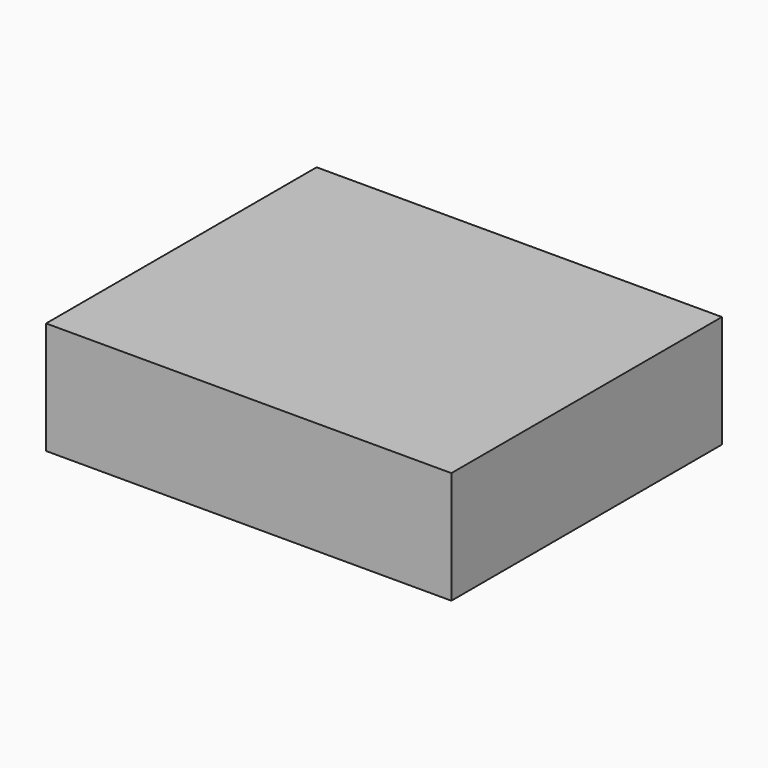
from build123d import *

# Parameters (mm, degrees)
F0_W     = 98.0573669076
F0_H     = 81.8147398531
F1_DEPTH = 27.178


# Not quite as in the source:
# - the program builds the solid bodies; features that only make, move or delete a surface that nothing else refers to are left out


with BuildPart() as f1:
    # F0 (on Top) → F1 (new body)
    with BuildSketch(Plane.XY):
        with Locations((3.4590773284, -6.7677628249)):
            Rectangle(F0_W, F0_H)
    extrude(amount=F1_DEPTH)


solid = f1.part
